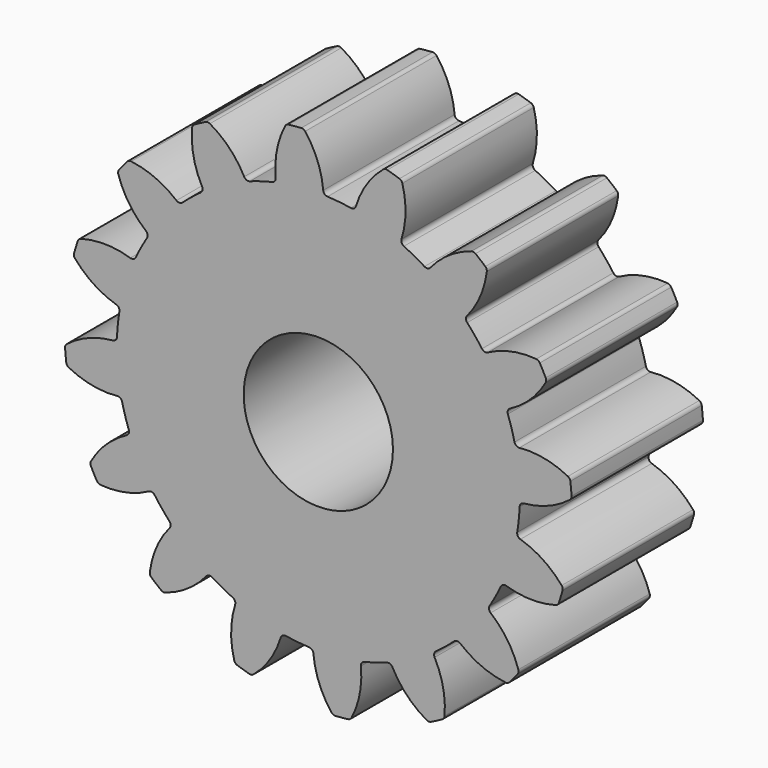
from build123d import *

# Parameters (mm, degrees)
F1_DEPTH = 2.2
F2_R     = 1
F3_DEPTH = 2.201


# Not quite as in the source:
# - a feature names something its author has since deleted; it is built from what else it names


with BuildPart() as f1:
    # F0 (on Front) → F1 (new body)
    with BuildSketch(Plane.XZ):
        with BuildLine():
            ThreePointArc((0.0658501888, 2.7527937353), (-0.0107962206, 3.0784970655), (-0.1768571825, 3.3689812963))
            ThreePointArc((-0.1768571825, 3.3689812963), (-0.2000460149, 3.3871150499), (-0.2290271151, 3.3922774917))
            ThreePointArc((-0.2290271151, 3.3922774917), (-0.3137124222, 3.3854961994), (-0.3982018601, 3.376601143))
            ThreePointArc((-0.3982018601, 3.376601143), (-0.4257409058, 3.3662013384), (-0.4452028358, 3.3441154096))
            ThreePointArc((-0.4452028358, 3.3441154096), (-0.5550599569, 3.0280636032), (-0.5705534857, 2.6938222503))
            ThreePointArc((-0.5705534857, 2.6938222503), (-0.5816569835, 2.6523658625), (-0.6173153418, 2.6284827884))
            ThreePointArc((-0.6173153418, 2.6284827884), (-0.7688345847, 2.5882220502), (-0.9177616204, 2.539234847))
            ThreePointArc((-0.9177616204, 2.539234847), (-1.258998717, 2.3884979026), (-1.5762018248, 2.1921650959))
            ThreePointArc((-1.5762018248, 2.1921650959), (-1.7007802346, 2.09698512), (-1.8196242836, 1.9947349364))
            ThreePointArc((-1.8196242836, 1.9947349364), (-2.0772017217, 1.7248863753), (-2.2951258682, 1.4221101396))
            ThreePointArc((-2.2951258682, 1.4221101396), (-2.3737975114, 1.2865012145), (-2.4444656446, 1.1465547141))
            ThreePointArc((-2.4444656446, 1.1465547141), (-2.5791695941, 0.7986765335), (-2.6646378036, 0.435551806))
            ThreePointArc((-2.6646378036, 0.435551806), (-2.6854256356, 0.2801591612), (-2.6971592704, 0.12382193))
            ThreePointArc((-2.6971592704, 0.12382193), (-2.688482276, -0.2491245706), (-2.6284827884, -0.6173153418))
            ThreePointArc((-2.6284827884, -0.6173153418), (-2.5882220502, -0.7688345847), (-2.539234847, -0.9177616204))
            ThreePointArc((-2.539234847, -0.9177616204), (-2.3884979026, -1.258998717), (-2.1921650959, -1.5762018248))
            ThreePointArc((-2.1921650959, -1.5762018248), (-2.09698512, -1.7007802346), (-1.9947349364, -1.8196242836))
            ThreePointArc((-1.9947349364, -1.8196242836), (-1.7248863753, -2.0772017217), (-1.4221101396, -2.2951258682))
            ThreePointArc((-1.4221101396, -2.2951258682), (-1.2865012145, -2.3737975114), (-1.1465547141, -2.4444656446))
            ThreePointArc((-1.1465547141, -2.4444656446), (-0.7986765335, -2.5791695941), (-0.435551806, -2.6646378036))
            ThreePointArc((-0.435551806, -2.6646378036), (-0.2801591612, -2.6854256356), (-0.12382193, -2.6971592704))
            ThreePointArc((-0.12382193, -2.6971592704), (0.2491245706, -2.688482276), (0.6173153418, -2.6284827884))
            ThreePointArc((0.6173153418, -2.6284827884), (0.7688345847, -2.5882220502), (0.9177616204, -2.539234847))
            ThreePointArc((0.9177616204, -2.539234847), (1.258998717, -2.3884979026), (1.5762018248, -2.1921650959))
            ThreePointArc((1.5762018248, -2.1921650959), (1.7007802346, -2.09698512), (1.8196242836, -1.9947349364))
            ThreePointArc((1.8196242836, -1.9947349364), (2.0772017217, -1.7248863753), (2.2951258682, -1.4221101396))
            ThreePointArc((2.2951258682, -1.4221101396), (2.3737975114, -1.2865012145), (2.4444656446, -1.1465547141))
            ThreePointArc((2.4444656446, -1.1465547141), (2.5791695941, -0.7986765335), (2.6646378036, -0.435551806))
            ThreePointArc((2.6646378036, -0.435551806), (2.6854256356, -0.2801591612), (2.6971592704, -0.12382193))
            ThreePointArc((2.6971592704, -0.12382193), (2.688482276, 0.2491245706), (2.6284827884, 0.6173153418))
            ThreePointArc((2.6284827884, 0.6173153418), (2.5882220502, 0.7688345847), (2.539234847, 0.9177616204))
            ThreePointArc((2.539234847, 0.9177616204), (2.3884979026, 1.258998717), (2.1921650959, 1.5762018248))
            ThreePointArc((2.1921650959, 1.5762018248), (2.09698512, 1.7007802346), (1.9947349364, 1.8196242836))
            ThreePointArc((1.9947349364, 1.8196242836), (1.7248863753, 2.0772017217), (1.4221101396, 2.2951258682))
            ThreePointArc((1.4221101396, 2.2951258682), (1.2865012145, 2.3737975114), (1.1465547141, 2.4444656446))
            ThreePointArc((1.1465547141, 2.4444656446), (0.7986765335, 2.5791695941), (0.435551806, 2.6646378036))
            ThreePointArc((0.435551806, 2.6646378036), (0.2801591612, 2.6854256356), (0.12382193, 2.6971592704))
            ThreePointArc((0.12382193, 2.6971592704), (0.0843822197, 2.7140834836), (0.0658501888, 2.7527937353))
        make_face()
        with BuildLine():
            ThreePointArc((-1.5762018248, 2.1921650959), (-1.258998717, 2.3884979026), (-0.9177616204, 2.539234847))
            ThreePointArc((-0.9177616204, 2.539234847), (-0.9606757776, 2.5397778575), (-0.9926109136, 2.5684495655))
            ThreePointArc((-0.9926109136, 2.5684495655), (-1.1880642308, 2.8400288949), (-1.4526480571, 3.0448525514))
            ThreePointArc((-1.4526480571, 3.0448525514), (-1.4810112319, 3.0527319733), (-1.5097618581, 3.0464108606))
            ThreePointArc((-1.5097618581, 3.0464108606), (-1.5854057918, 3.0077380995), (-1.6600598635, 2.9671874308))
            ThreePointArc((-1.6600598635, 2.9671874308), (-1.6815227913, 2.9470405277), (-1.691051351, 2.9191880319))
            ThreePointArc((-1.691051351, 2.9191880319), (-1.6715983066, 2.5851537366), (-1.5580038326, 2.270425875))
            ThreePointArc((-1.5580038326, 2.270425875), (-1.5523974541, 2.2278760422), (-1.5762018248, 2.1921650959))
        make_face()
        with BuildLine():
            ThreePointArc((-2.2951258682, 1.4221101396), (-2.0772017217, 1.7248863753), (-1.8196242836, 1.9947349364))
            ThreePointArc((-1.8196242836, 1.9947349364), (-1.8594795962, 1.9788140757), (-1.8999560024, 1.9930822324))
            ThreePointArc((-1.8999560024, 1.9930822324), (-2.1844602317, 2.1691920701), (-2.5072864333, 2.2571726072))
            ThreePointArc((-2.5072864333, 2.2571726072), (-2.5365059142, 2.2535981268), (-2.5606490442, 2.2367557919))
            ThreePointArc((-2.5606490442, 2.2367557919), (-2.6157355013, 2.1720791392), (-2.6691888011, 2.10604633))
            ThreePointArc((-2.6691888011, 2.10604633), (-2.6813080748, 2.0792195117), (-2.6794526274, 2.049840739))
            ThreePointArc((-2.6794526274, 2.049840739), (-2.5336509672, 1.7486776481), (-2.3082622193, 1.5013777417))
            ThreePointArc((-2.3082622193, 1.5013777417), (-2.2867994849, 1.4642122902), (-2.2951258682, 1.4221101396))
        make_face()
        with BuildLine():
            ThreePointArc((-2.6646378036, 0.435551806), (-2.5791695941, 0.7986765335), (-2.4444656446, 1.1465547141))
            ThreePointArc((-2.4444656446, 1.1465547141), (-2.4751945026, 1.1165937889), (-2.518050013, 1.1142861968))
            ThreePointArc((-2.518050013, 1.1142861968), (-2.8482919645, 1.1681154163), (-3.1802131787, 1.1258585949))
            ThreePointArc((-3.1802131787, 1.1258585949), (-3.2058405645, 1.1113743944), (-3.2217006257, 1.08657493))
            ThreePointArc((-3.2217006257, 1.08657493), (-3.2478431925, 1.0057408199), (-3.27195794, 0.9242787667))
            ThreePointArc((-3.27195794, 0.9242787667), (-3.27288851, 0.8948561732), (-3.2599315306, 0.8684237753))
            ThreePointArc((-3.2599315306, 0.8684237753), (-3.0099782356, 0.6459812395), (-2.7071086075, 0.5037584573))
            ThreePointArc((-2.7071086075, 0.5037584573), (-2.673057024, 0.4776354902), (-2.6646378036, 0.435551806))
        make_face()
        with BuildLine():
            ThreePointArc((-2.6284827884, -0.6173153418), (-2.688482276, -0.2491245706), (-2.6971592704, 0.12382193))
            ThreePointArc((-2.6971592704, 0.12382193), (-2.7140834836, 0.0843822197), (-2.7527937353, 0.0658501888))
            ThreePointArc((-2.7527937353, 0.0658501888), (-3.0784970655, -0.0107962206), (-3.3689812963, -0.1768571825))
            ThreePointArc((-3.3689812963, -0.1768571825), (-3.3871150499, -0.2000460149), (-3.3922774917, -0.2290271151))
            ThreePointArc((-3.3922774917, -0.2290271151), (-3.3854961994, -0.3137124222), (-3.376601143, -0.3982018601))
            ThreePointArc((-3.376601143, -0.3982018601), (-3.3662013384, -0.4257409058), (-3.3441154096, -0.4452028358))
            ThreePointArc((-3.3441154096, -0.4452028358), (-3.0280636032, -0.5550599569), (-2.6938222503, -0.5705534857))
            ThreePointArc((-2.6938222503, -0.5705534857), (-2.6523658625, -0.5816569835), (-2.6284827884, -0.6173153418))
        make_face()
        with BuildLine():
            ThreePointArc((0.5037584573, 2.7071086075), (0.4776354902, 2.673057024), (0.435551806, 2.6646378036))
            ThreePointArc((0.435551806, 2.6646378036), (0.7986765335, 2.5791695941), (1.1465547141, 2.4444656446))
            ThreePointArc((1.1465547141, 2.4444656446), (1.1165937889, 2.4751945026), (1.1142861968, 2.518050013))
            ThreePointArc((1.1142861968, 2.518050013), (1.1681154163, 2.8482919645), (1.1258585949, 3.1802131787))
            ThreePointArc((1.1258585949, 3.1802131787), (1.1113743944, 3.2058405645), (1.08657493, 3.2217006257))
            ThreePointArc((1.08657493, 3.2217006257), (1.0057408199, 3.2478431925), (0.9242787667, 3.27195794))
            ThreePointArc((0.9242787667, 3.27195794), (0.8948561732, 3.27288851), (0.8684237753, 3.2599315306))
            ThreePointArc((0.8684237753, 3.2599315306), (0.6459812395, 3.0099782356), (0.5037584573, 2.7071086075))
        make_face()
        with BuildLine():
            ThreePointArc((1.5013777417, 2.3082622193), (1.4642122902, 2.2867994849), (1.4221101396, 2.2951258682))
            ThreePointArc((1.4221101396, 2.2951258682), (1.7248863753, 2.0772017217), (1.9947349364, 1.8196242836))
            ThreePointArc((1.9947349364, 1.8196242836), (1.9788140757, 1.8594795962), (1.9930822324, 1.8999560024))
            ThreePointArc((1.9930822324, 1.8999560024), (2.1691920701, 2.1844602317), (2.2571726072, 2.5072864333))
            ThreePointArc((2.2571726072, 2.5072864333), (2.2535981268, 2.5365059142), (2.2367557919, 2.5606490442))
            ThreePointArc((2.2367557919, 2.5606490442), (2.1720791392, 2.6157355013), (2.10604633, 2.6691888011))
            ThreePointArc((2.10604633, 2.6691888011), (2.0792195117, 2.6813080748), (2.049840739, 2.6794526274))
            ThreePointArc((2.049840739, 2.6794526274), (1.7486776481, 2.5336509672), (1.5013777417, 2.3082622193))
        make_face()
        with BuildLine():
            ThreePointArc((2.270425875, 1.5580038326), (2.2278760422, 1.5523974541), (2.1921650959, 1.5762018248))
            ThreePointArc((2.1921650959, 1.5762018248), (2.3884979026, 1.258998717), (2.539234847, 0.9177616204))
            ThreePointArc((2.539234847, 0.9177616204), (2.5397778575, 0.9606757776), (2.5684495655, 0.9926109136))
            ThreePointArc((2.5684495655, 0.9926109136), (2.8400288949, 1.1880642308), (3.0448525514, 1.4526480571))
            ThreePointArc((3.0448525514, 1.4526480571), (3.0527319733, 1.4810112319), (3.0464108606, 1.5097618581))
            ThreePointArc((3.0464108606, 1.5097618581), (3.0077380995, 1.5854057918), (2.9671874308, 1.6600598635))
            ThreePointArc((2.9671874308, 1.6600598635), (2.9470405277, 1.6815227913), (2.9191880319, 1.691051351))
            ThreePointArc((2.9191880319, 1.691051351), (2.5851537366, 1.6715983066), (2.270425875, 1.5580038326))
        make_face()
        with BuildLine():
            ThreePointArc((2.6938222503, 0.5705534857), (2.6523658625, 0.5816569835), (2.6284827884, 0.6173153418))
            ThreePointArc((2.6284827884, 0.6173153418), (2.688482276, 0.2491245706), (2.6971592704, -0.12382193))
            ThreePointArc((2.6971592704, -0.12382193), (2.7140834836, -0.0843822197), (2.7527937353, -0.0658501888))
            ThreePointArc((2.7527937353, -0.0658501888), (3.0784970655, 0.0107962206), (3.3689812963, 0.1768571825))
            ThreePointArc((3.3689812963, 0.1768571825), (3.3871150499, 0.2000460149), (3.3922774917, 0.2290271151))
            ThreePointArc((3.3922774917, 0.2290271151), (3.3854961994, 0.3137124222), (3.376601143, 0.3982018601))
            ThreePointArc((3.376601143, 0.3982018601), (3.3662013384, 0.4257409058), (3.3441154096, 0.4452028358))
            ThreePointArc((3.3441154096, 0.4452028358), (3.0280636032, 0.5550599569), (2.6938222503, 0.5705534857))
        make_face()
        with BuildLine():
            ThreePointArc((2.7071086075, -0.5037584573), (2.673057024, -0.4776354902), (2.6646378036, -0.435551806))
            ThreePointArc((2.6646378036, -0.435551806), (2.5791695941, -0.7986765335), (2.4444656446, -1.1465547141))
            ThreePointArc((2.4444656446, -1.1465547141), (2.4751945026, -1.1165937889), (2.518050013, -1.1142861968))
            ThreePointArc((2.518050013, -1.1142861968), (2.8482919645, -1.1681154163), (3.1802131787, -1.1258585949))
            ThreePointArc((3.1802131787, -1.1258585949), (3.2058405645, -1.1113743944), (3.2217006257, -1.08657493))
            ThreePointArc((3.2217006257, -1.08657493), (3.2478431925, -1.0057408199), (3.27195794, -0.9242787667))
            ThreePointArc((3.27195794, -0.9242787667), (3.27288851, -0.8948561732), (3.2599315306, -0.8684237753))
            ThreePointArc((3.2599315306, -0.8684237753), (3.0099782356, -0.6459812395), (2.7071086075, -0.5037584573))
        make_face()
        with BuildLine():
            ThreePointArc((2.3082622193, -1.5013777417), (2.2867994849, -1.4642122902), (2.2951258682, -1.4221101396))
            ThreePointArc((2.2951258682, -1.4221101396), (2.0772017217, -1.7248863753), (1.8196242836, -1.9947349364))
            ThreePointArc((1.8196242836, -1.9947349364), (1.8594795962, -1.9788140757), (1.8999560024, -1.9930822324))
            ThreePointArc((1.8999560024, -1.9930822324), (2.1844602317, -2.1691920701), (2.5072864333, -2.2571726072))
            ThreePointArc((2.5072864333, -2.2571726072), (2.5365059142, -2.2535981268), (2.5606490442, -2.2367557919))
            ThreePointArc((2.5606490442, -2.2367557919), (2.6157355013, -2.1720791392), (2.6691888011, -2.10604633))
            ThreePointArc((2.6691888011, -2.10604633), (2.6813080748, -2.0792195117), (2.6794526274, -2.049840739))
            ThreePointArc((2.6794526274, -2.049840739), (2.5336509672, -1.7486776481), (2.3082622193, -1.5013777417))
        make_face()
        with BuildLine():
            ThreePointArc((1.5580038326, -2.270425875), (1.5523974541, -2.2278760422), (1.5762018248, -2.1921650959))
            ThreePointArc((1.5762018248, -2.1921650959), (1.258998717, -2.3884979026), (0.9177616204, -2.539234847))
            ThreePointArc((0.9177616204, -2.539234847), (0.9606757776, -2.5397778575), (0.9926109136, -2.5684495655))
            ThreePointArc((0.9926109136, -2.5684495655), (1.1880642308, -2.8400288949), (1.4526480571, -3.0448525514))
            ThreePointArc((1.4526480571, -3.0448525514), (1.4810112319, -3.0527319733), (1.5097618581, -3.0464108606))
            ThreePointArc((1.5097618581, -3.0464108606), (1.5854057918, -3.0077380995), (1.6600598635, -2.9671874308))
            ThreePointArc((1.6600598635, -2.9671874308), (1.6815227913, -2.9470405277), (1.691051351, -2.9191880319))
            ThreePointArc((1.691051351, -2.9191880319), (1.6715983066, -2.5851537366), (1.5580038326, -2.270425875))
        make_face()
        with BuildLine():
            ThreePointArc((0.5705534857, -2.6938222503), (0.5816569835, -2.6523658625), (0.6173153418, -2.6284827884))
            ThreePointArc((0.6173153418, -2.6284827884), (0.2491245706, -2.688482276), (-0.12382193, -2.6971592704))
            ThreePointArc((-0.12382193, -2.6971592704), (-0.0843822197, -2.7140834836), (-0.0658501888, -2.7527937353))
            ThreePointArc((-0.0658501888, -2.7527937353), (0.0107962206, -3.0784970655), (0.1768571825, -3.3689812963))
            ThreePointArc((0.1768571825, -3.3689812963), (0.2000460149, -3.3871150499), (0.2290271151, -3.3922774917))
            ThreePointArc((0.2290271151, -3.3922774917), (0.3137124222, -3.3854961994), (0.3982018601, -3.376601143))
            ThreePointArc((0.3982018601, -3.376601143), (0.4257409058, -3.3662013384), (0.4452028358, -3.3441154096))
            ThreePointArc((0.4452028358, -3.3441154096), (0.5550599569, -3.0280636032), (0.5705534857, -2.6938222503))
        make_face()
        with BuildLine():
            ThreePointArc((-0.435551806, -2.6646378036), (-0.7986765335, -2.5791695941), (-1.1465547141, -2.4444656446))
            ThreePointArc((-1.1465547141, -2.4444656446), (-1.1165937889, -2.4751945026), (-1.1142861968, -2.518050013))
            ThreePointArc((-1.1142861968, -2.518050013), (-1.1681154163, -2.8482919645), (-1.1258585949, -3.1802131787))
            ThreePointArc((-1.1258585949, -3.1802131787), (-1.1113743944, -3.2058405645), (-1.08657493, -3.2217006257))
            ThreePointArc((-1.08657493, -3.2217006257), (-1.0057408199, -3.2478431925), (-0.9242787667, -3.27195794))
            ThreePointArc((-0.9242787667, -3.27195794), (-0.8948561732, -3.27288851), (-0.8684237753, -3.2599315306))
            ThreePointArc((-0.8684237753, -3.2599315306), (-0.6459812395, -3.0099782356), (-0.5037584573, -2.7071086075))
            ThreePointArc((-0.5037584573, -2.7071086075), (-0.4776354902, -2.673057024), (-0.435551806, -2.6646378036))
        make_face()
        with BuildLine():
            ThreePointArc((-1.4221101396, -2.2951258682), (-1.7248863753, -2.0772017217), (-1.9947349364, -1.8196242836))
            ThreePointArc((-1.9947349364, -1.8196242836), (-1.9788140757, -1.8594795962), (-1.9930822324, -1.8999560024))
            ThreePointArc((-1.9930822324, -1.8999560024), (-2.1691920701, -2.1844602317), (-2.2571726072, -2.5072864333))
            ThreePointArc((-2.2571726072, -2.5072864333), (-2.2535981268, -2.5365059142), (-2.2367557919, -2.5606490442))
            ThreePointArc((-2.2367557919, -2.5606490442), (-2.1720791392, -2.6157355013), (-2.10604633, -2.6691888011))
            ThreePointArc((-2.10604633, -2.6691888011), (-2.0792195117, -2.6813080748), (-2.049840739, -2.6794526274))
            ThreePointArc((-2.049840739, -2.6794526274), (-1.7486776481, -2.5336509672), (-1.5013777417, -2.3082622193))
            ThreePointArc((-1.5013777417, -2.3082622193), (-1.4642122902, -2.2867994849), (-1.4221101396, -2.2951258682))
        make_face()
        with BuildLine():
            ThreePointArc((-2.1921650959, -1.5762018248), (-2.3884979026, -1.258998717), (-2.539234847, -0.9177616204))
            ThreePointArc((-2.539234847, -0.9177616204), (-2.5397778575, -0.9606757776), (-2.5684495655, -0.9926109136))
            ThreePointArc((-2.5684495655, -0.9926109136), (-2.8400288949, -1.1880642308), (-3.0448525514, -1.4526480571))
            ThreePointArc((-3.0448525514, -1.4526480571), (-3.0527319733, -1.4810112319), (-3.0464108606, -1.5097618581))
            ThreePointArc((-3.0464108606, -1.5097618581), (-3.0077380995, -1.5854057918), (-2.9671874308, -1.6600598635))
            ThreePointArc((-2.9671874308, -1.6600598635), (-2.9470405277, -1.6815227913), (-2.9191880319, -1.691051351))
            ThreePointArc((-2.9191880319, -1.691051351), (-2.5851537366, -1.6715983066), (-2.270425875, -1.5580038326))
            ThreePointArc((-2.270425875, -1.5580038326), (-2.2278760422, -1.5523974541), (-2.1921650959, -1.5762018248))
        make_face()
    extrude(amount=F1_DEPTH)

    # F2 (on face) → F3 (cut, through all)
    with BuildSketch(Plane.XZ.offset(2.2)):
        Circle(F2_R)
    extrude(amount=-F3_DEPTH, mode=Mode.SUBTRACT)


solid = f1.part
